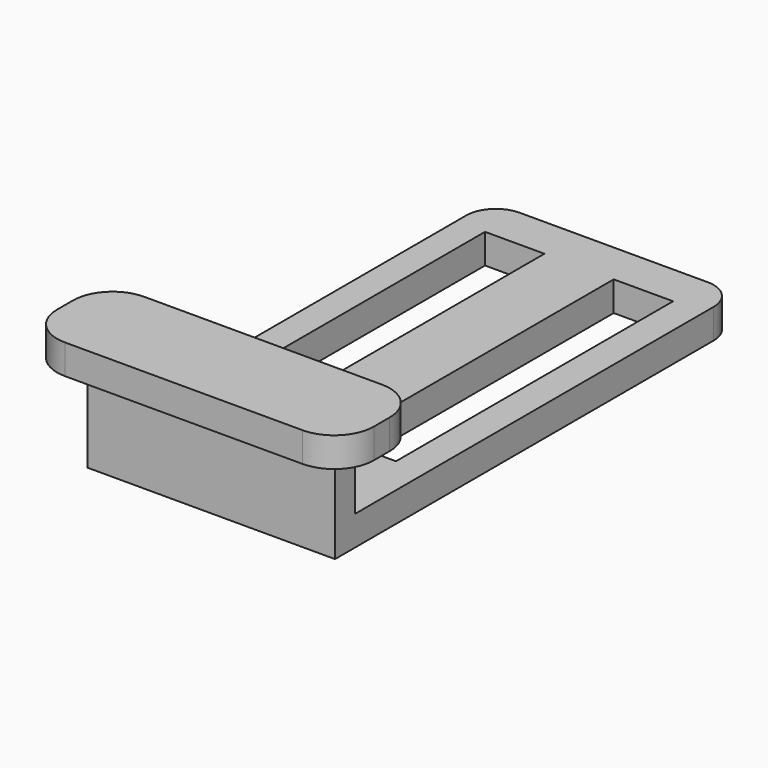
from build123d import *

# Parameters (mm, degrees)
F0_W     = 25
F0_H     = 3.598708484
F0_H_2   = 2.5
F0_H_3   = 44.7172746155
F0_W_2   = 6
F0_H_4   = 35
F1_DEPTH = 3
F2_DEPTH = 10
F3_START = 10
F3_DEPTH = 3
F4_R     = 4
F5_R     = 3


# Not quite as in the source:
# - a feature names something its author has since deleted; it is built from what else it names


with BuildPart() as f1:
    # F0 (on Top) → F1 (new body)
    with BuildSketch(Plane.XY):
        with Locations((0.1855289564, 2.9724632242)):
            Rectangle(F0_W, F0_H)
        with Locations((0.1855289564, -0.0768910178)):
            Rectangle(F0_W, F0_H_2)
        with Locations((0.1855289564, 27.130454774)):
            Rectangle(F0_W, F0_H_3)
        with Locations((-6.4080492333, 27.7351317182)):
            Rectangle(F0_W_2, F0_H_4, mode=Mode.SUBTRACT)
        with Locations((6.5919507667, 27.7351317182)):
            Rectangle(F0_W_2, F0_H_4, mode=Mode.SUBTRACT)
    extrude(amount=F1_DEPTH)

    # F0 (on Top) → F2 (join)
    with BuildSketch(Plane.XY):
        with Locations((0.1855289564, -0.0768910178)):
            Rectangle(F0_W, F0_H_2)
    extrude(amount=F2_DEPTH)

    # F0 (on Top) → F3 (join)
    with BuildSketch(Plane.XY.offset(F3_START)):
        with Locations((0.1855289564, 2.9724632242)):
            Rectangle(F0_W, F0_H)
        Polygon((-12.3144710436, -1.3268910178), (-12.3144710436, 1.1731089822), (-12.3144710436, 4.7718174662), (-15.4697376937, 4.7718174662), (-15.4697376937, -5.2281825338), (16.5302623063, -5.2281825338), (16.5302623063, 4.7718174662), (12.6855289564, 4.7718174662), (12.6855289564, 1.1731089822), (12.6855289564, -1.3268910178), align=None)
        with Locations((0.1855289564, -0.0768910178)):
            Rectangle(F0_W, F0_H_2)
    extrude(amount=F3_DEPTH)

    # F4
    f4_edges = [f1.edges().sort_by_distance(p)[0] for p in [
        (16.530262, -5.228183, 11.5),
        (16.530262, 4.771817, 11.5),
        (-15.469738, -5.228183, 11.5),
        (-15.469738, 4.771817, 11.5),
    ]]
    fillet(f4_edges, radius=F4_R)

    # F5
    f5_edges = [f1.edges().sort_by_distance(p)[0] for p in [
        (-12.314471, 49.489092, 1.5),
        (12.685529, 49.489092, 1.5),
    ]]
    fillet(f5_edges, radius=F5_R)


solid = f1.part
